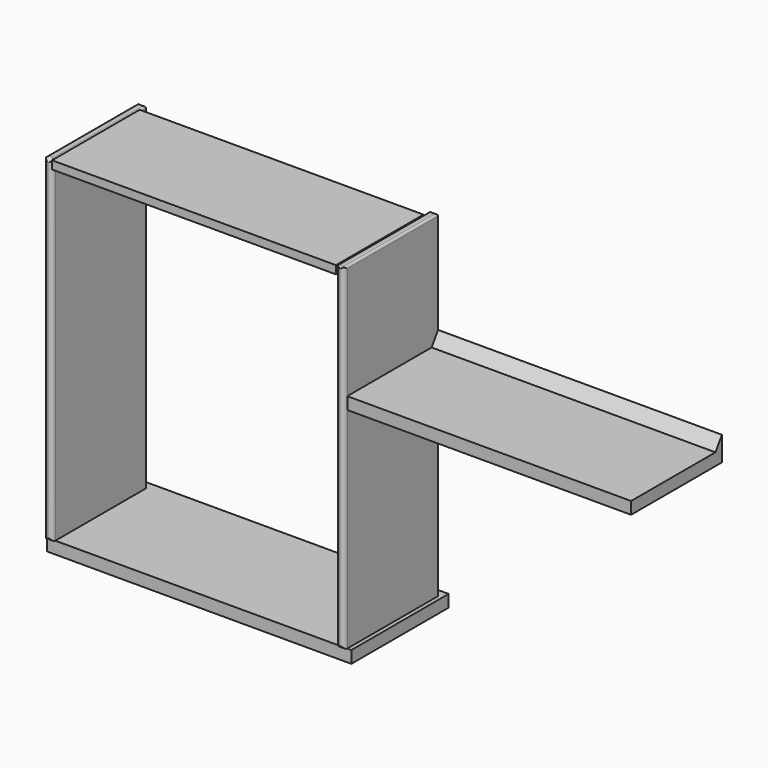
from build123d import *

# Parameters (mm, degrees)
F0_W        = 368.3
F0_H        = 1054.1
F1_DEPTH    = 25.4
F2_R        = 6.35
F3_T1_DEPTH = 1111.25
F3_T3_DEPTH = 88.9
F4_W        = 889
F4_H        = 342.9
F5_DEPTH    = 25.4
F6_W        = 368.3
F6_H        = 1054.1
F7_DEPTH    = 25.4
F8_R        = 12.69999
F9_T1_DEPTH = 387.35001
F9_T3_DEPTH = 57.15
F11_DEPTH   = 889
F12_W       = 952.5
F12_H       = 381
F13_DEPTH   = 38.1


# Not quite as in the source:
# - a fillet or chamfer that OpenCascade refuses, or shapes differently, is made with other operations: its cross-section is extruded or revolved along the edge and cut away or added
# - a fillet or chamfer is up to 0.001 mm smaller than in the source, because OpenCascade refuses the exact size


with BuildPart() as f1:
    # F0 (on Right) → F1 (new body)
    with BuildSketch(Plane.YZ):
        with Locations((184.15, -527.05)):
            Rectangle(F0_W, F0_H)
    extrude(amount=F1_DEPTH)

    # F2
    f2_edges = [f1.edges().sort_by_distance(p)[0] for p in [
        (12.7, 368.3, 0),
        (12.7, 0, 0),
        (0, 184.15, 0),
        (25.4, 184.15, 0),
    ]]
    fillet(f2_edges, radius=F2_R)

    # F3: fillet of radius 12.7 on 4 edges, made by hand

    # F3_s2 → F3_t1 (cut)
    with BuildSketch(Plane.XY.offset(-1085.85)):
        with BuildLine():
            ThreePointArc((0, 12.7), (3.7197438789, 3.7197438789), (12.7, 0))
            Line((12.7, 0), (0, 0))
            Line((0, 0), (0, 12.7))
        make_face()
        with BuildLine():
            ThreePointArc((25.4, 12.7), (21.6802561211, 3.7197438789), (12.7, 0))
            Line((12.7, 0), (25.4, 0))
            Line((25.4, 0), (25.4, 12.7))
        make_face()
    extrude(amount=F3_T1_DEPTH, mode=Mode.SUBTRACT)

    # F3_s4 → F3_t3 (cut)
    with BuildSketch(Plane.YZ.offset(-31.75)):
        with BuildLine():
            ThreePointArc((0, -1041.4), (3.7197438789, -1050.3802561211), (12.7, -1054.1))
            Line((12.7, -1054.1), (0, -1054.1))
            Line((0, -1054.1), (0, -1041.4))
        make_face()
    extrude(amount=F3_T3_DEPTH, mode=Mode.SUBTRACT)


with BuildPart() as f5:
    # F4 (on Top) → F5 (new body)
    with BuildSketch(Plane.XY):
        with Locations((-444.5, 171.45)):
            Rectangle(F4_W, F4_H)
    extrude(amount=-F5_DEPTH)


with BuildPart() as f7:
    # F6 (on face) → F7 (new body)
    with BuildSketch(Plane(origin=(-889, 0, 0), x_dir=(0, -1, 0), z_dir=(-1, 0, 0))):
        with Locations((-184.15, -527.05)):
            Rectangle(F6_W, F6_H)
    extrude(amount=F7_DEPTH)

    # F8 (radius 12.7 in the source; OpenCascade refuses exactly that, so slightly less here)
    f8_edges = [f7.edges().sort_by_distance(p)[0] for p in [
        (-901.7, 0, -1054.1),
        (-901.7, 0, 0),
        (-889, 0, -527.05),
        (-914.4, 0, -527.05),
    ]]
    fillet(f8_edges, radius=F8_R)

    # F9: fillet of radius 6.35 on 4 edges, made by hand

    # F9_s2 → F9_t1 (cut)
    with BuildSketch(Plane.XZ.offset(-384.175)):
        with BuildLine():
            ThreePointArc((-889, -6.35), (-890.8598719395, -1.8598719395), (-895.35, 0))
            Line((-895.35, 0), (-889, 0))
            Line((-889, 0), (-889, -6.35))
        make_face()
        with BuildLine():
            ThreePointArc((-914.4, -6.35), (-912.5401280605, -1.8598719395), (-908.05, 0))
            Line((-908.05, 0), (-914.4, 0))
            Line((-914.4, 0), (-914.4, -6.35))
        make_face()
    extrude(amount=F9_T1_DEPTH, mode=Mode.SUBTRACT)

    # F9_s4 → F9_t3 (cut)
    with BuildSketch(Plane.YZ.offset(-930.275)):
        with BuildLine():
            ThreePointArc((361.95, 0), (366.4401280605, -1.8598719395), (368.3, -6.35))
            Line((368.3, -6.35), (368.3, 0))
            Line((368.3, 0), (361.95, 0))
        make_face()
    extrude(amount=F9_T3_DEPTH, mode=Mode.SUBTRACT)


with BuildPart() as f11:
    # F10 (on face) → F11 (new body)
    with BuildSketch(Plane.YZ.offset(25.4)):
        Polygon((368.3, -396.2427675724), (368.3, -320.0427675724), (342.9, -358.1427675724), (12.7, -358.1427675724), (12.7, -396.2427675724), align=None)
    extrude(amount=F11_DEPTH)


with BuildPart() as f13:
    # F12 (on face) → F13 (new body)
    with BuildSketch(Plane(origin=(0, 0, -1054.1), x_dir=(1, 0, 0), z_dir=(0, 0, -1))):
        with Locations((-438.15, -203.2)):
            Rectangle(F12_W, F12_H)
    extrude(amount=F13_DEPTH)


solid = Compound([f1.part, f5.part, f7.part, f11.part, f13.part])
